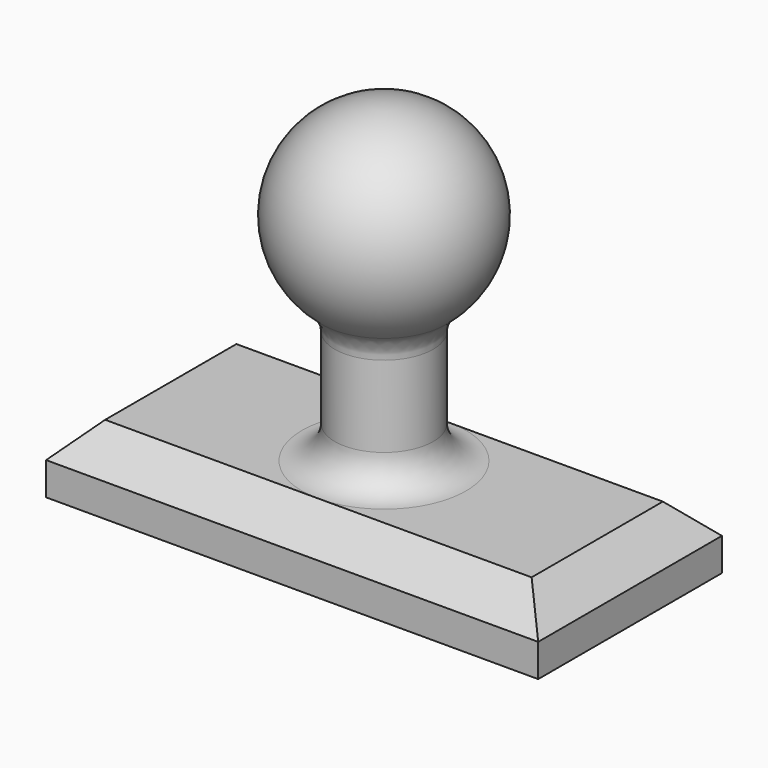
from build123d import *

# Parameters (mm, degrees)
F2_W     = 15
F2_H     = 7
F2_R     = 1.5
F3_DEPTH = 2.000000095
F4_R     = 1
F5_SIZE  = 0.99999


# Not quite as in the source:
# - a fillet or chamfer is up to 0.001 mm smaller than in the source, because OpenCascade refuses the exact size


with BuildPart() as f1:
    # F0 (on Front) → F1 (revolve)
    with BuildSketch(Plane.XZ):
        with BuildLine():
            Line((-1.5, 4), (-1.5, 0))
            Line((-1.5, 0), (0, 0))
            Line((0, 0), (0, 9.5980762114))
            ThreePointArc((0, 9.5980762114), (-2.8977774789, 7.3745333467), (-1.5, 4))
        make_face()
    revolve(axis=Axis((0, 0, 4.7990381057), (0, 0, 1)))

    # F2 (on face) → F3 (join)
    with BuildSketch(Plane(origin=(0, 0, 0), x_dir=(1, 0, 0), z_dir=(0, 0, -1))):
        Rectangle(F2_W, F2_H)
        Circle(F2_R, mode=Mode.SUBTRACT)
        Circle(F2_R)
    extrude(amount=F3_DEPTH)

    # F4
    f4_edges = [f1.edges().sort_by_distance(p)[0] for p in [
        (1.5, 0, 0),
        (1.5, 0, 4),
    ]]
    fillet(f4_edges, radius=F4_R)

    # F5 (size 1 in the source; OpenCascade refuses exactly that, so slightly less here)
    f5_edges = [f1.edges().sort_by_distance(p)[0] for p in [
        (2.5, 0, 0),
        (7.5, 0, 0),
        (0, 3.5, 0),
        (0, -3.5, 0),
        (-7.5, 0, 0),
    ]]
    chamfer(f5_edges, length=F5_SIZE)


solid = f1.part
